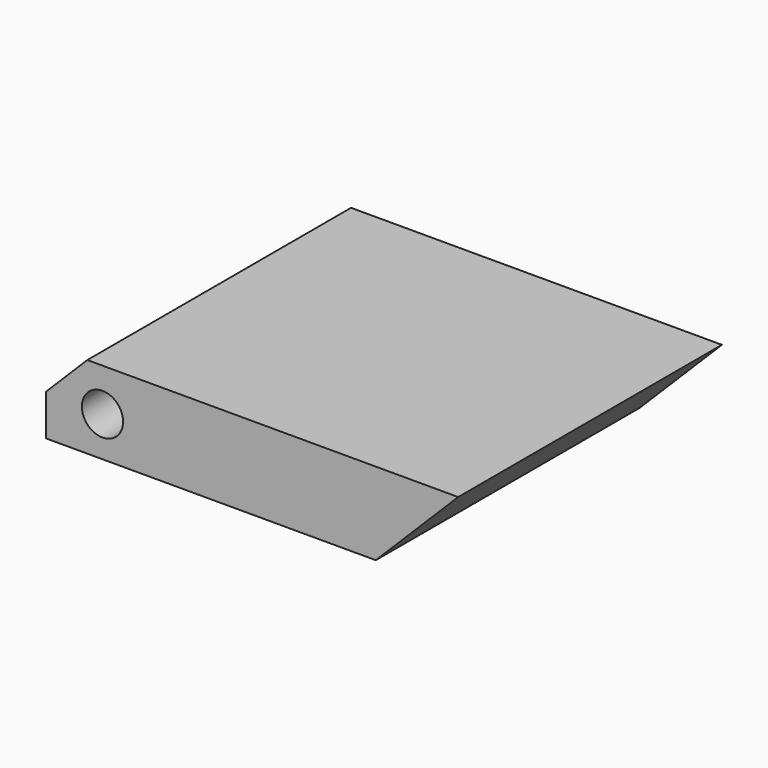
from build123d import *

# Parameters (mm, degrees)
F0_W     = 127
F0_H     = 25.4
F0_R     = 6.35
F1_DEPTH = 101.6
F2_SIZE  = 25.39999
F3_SIZE  = 12.7


# Not quite as in the source:
# - a fillet or chamfer is up to 0.001 mm smaller than in the source, because OpenCascade refuses the exact size


with BuildPart() as f1:
    # F0 (on Front) → F1 (new body)
    with BuildSketch(Plane.XZ):
        with Locations((5.6473743348, 0.4580724053)):
            Rectangle(F0_W, F0_H)
        with Locations((-40.4630713165, 0)):
            Circle(F0_R, mode=Mode.SUBTRACT)
    extrude(amount=-F1_DEPTH)

    # F2 (size 25.4 in the source; OpenCascade refuses exactly that, so slightly less here)
    f2_edges = [f1.edges().sort_by_distance(p)[0] for p in [
        (69.147374, 50.8, -12.241928),
    ]]
    chamfer(f2_edges, length=F2_SIZE)

    # F3
    f3_edges = [f1.edges().sort_by_distance(p)[0] for p in [
        (-57.852626, 50.8, 13.158072),
    ]]
    chamfer(f3_edges, length=F3_SIZE)


solid = f1.part
